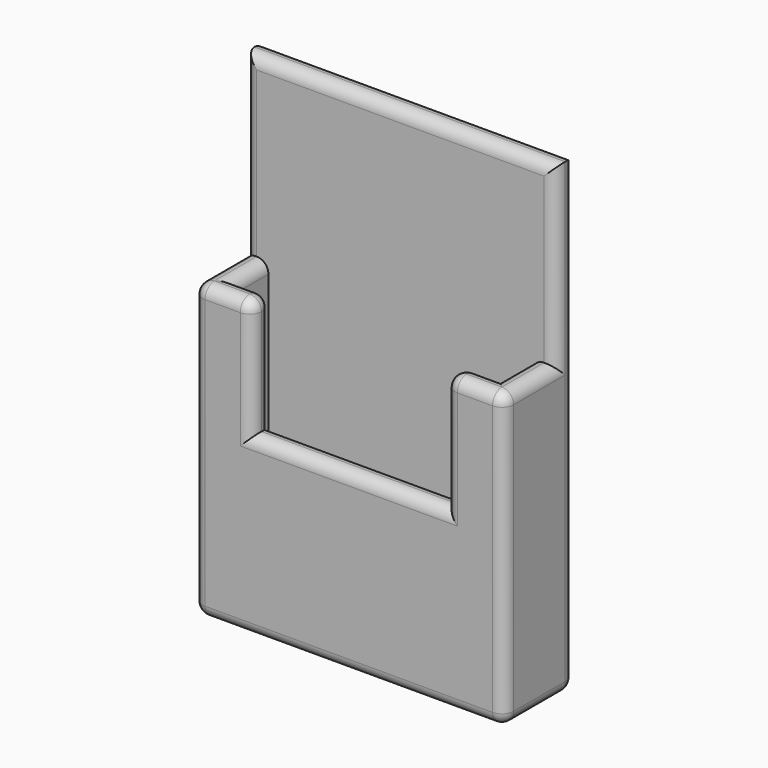
from build123d import *

# Parameters (mm, degrees)
F0_W     = 41.91
F0_H     = 5.08
F1_DEPTH = 5.08
F2_DEPTH = 101.6
F3_DEPTH = 63.5
F4_DEPTH = 38.1
F5_R     = 2.53999


# Not quite as in the source:
# - a fillet or chamfer is up to 0.001 mm smaller than in the source, because OpenCascade refuses the exact size


with BuildPart() as f1:
    # F0 (on Top) → F1 (new body)
    with BuildSketch(Plane.XY):
        Polygon((33.655, 9.525), (-33.655, 9.525), (-33.655, 4.445), (-28.575, 4.445), (28.575, 4.445), (33.655, 4.445), align=None)
        Polygon((-28.575, 4.445), (-33.655, 4.445), (-33.655, -9.525), (-20.955, -9.525), (-20.955, -4.445), (-28.575, -4.445), align=None)
        Polygon((33.655, -9.525), (33.655, 4.445), (28.575, 4.445), (28.575, -4.445), (20.955, -4.445), (20.955, -9.525), align=None)
        with Locations((0, -6.985)):
            Rectangle(F0_W, F0_H)
        Polygon((28.575, 4.445), (-28.575, 4.445), (-28.575, -4.445), (-20.955, -4.445), (20.955, -4.445), (28.575, -4.445), align=None)
    extrude(amount=F1_DEPTH)

    # F0 (on Top) → F2 (join)
    with BuildSketch(Plane.XY):
        Polygon((33.655, 9.525), (-33.655, 9.525), (-33.655, 4.445), (-28.575, 4.445), (28.575, 4.445), (33.655, 4.445), align=None)
    extrude(amount=F2_DEPTH)

    # F0 (on Top) → F3 (join)
    with BuildSketch(Plane.XY):
        Polygon((-28.575, 4.445), (-33.655, 4.445), (-33.655, -9.525), (-20.955, -9.525), (-20.955, -4.445), (-28.575, -4.445), align=None)
        Polygon((33.655, -9.525), (33.655, 4.445), (28.575, 4.445), (28.575, -4.445), (20.955, -4.445), (20.955, -9.525), align=None)
    extrude(amount=F3_DEPTH)

    # F0 (on Top) → F4 (join)
    with BuildSketch(Plane.XY):
        with Locations((0, -6.985)):
            Rectangle(F0_W, F0_H)
    extrude(amount=F4_DEPTH)

    # F5 (radius 2.54 in the source; OpenCascade refuses exactly that, so slightly less here)
    f5_edges = [f1.edges().sort_by_distance(p)[0] for p in [
        (-33.655, 4.445, 82.55),
        (33.655, 9.525, 50.8),
        (33.655, 4.445, 82.55),
        (0, 4.445, 101.6),
        (0, 9.525, 101.6),
        (-33.655, 9.525, 50.8),
        (0, 9.525, 0),
        (33.655, -2.54, 63.5),
        (24.765, -4.445, 63.5),
        (28.575, 0, 63.5),
        (27.305, -9.525, 63.5),
        (20.955, -6.985, 63.5),
        (33.655, -9.525, 31.75),
        (20.955, -9.525, 50.8),
        (0, -9.525, 38.1),
        (-20.955, -9.525, 50.8),
        (-20.955, -4.445, 50.8),
        (-27.305, -9.525, 63.5),
        (-24.765, -4.445, 63.5),
        (-28.575, 0, 63.5),
        (-33.655, -2.54, 63.5),
        (-33.655, -9.525, 31.75),
        (0, -9.525, 0),
        (33.655, 0, 0),
        (-33.655, 0, 0),
        (-20.955, -6.985, 63.5),
        (0, -4.445, 38.1),
        (20.955, -4.445, 50.8),
    ]]
    fillet(f5_edges, radius=F5_R)


solid = f1.part
